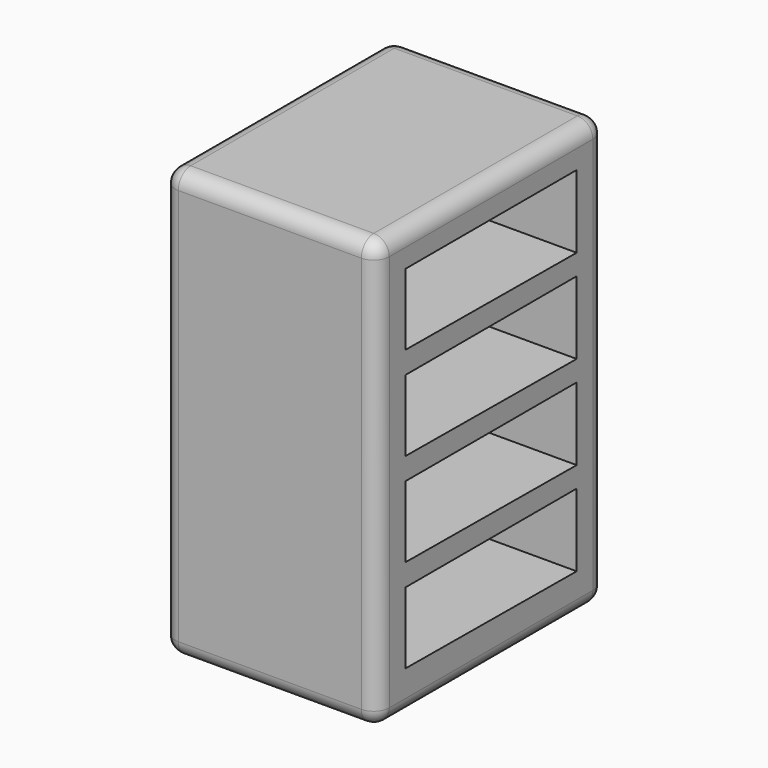
from build123d import *

# Parameters (mm, degrees)
F0_W     = 76.2
F0_H     = 101.6
F1_DEPTH = 152.4
F3_DEPTH = 50.8
F4_R     = 5.5188922036


# Not quite as in the source:
# - a feature names something its author has since deleted; it is built from what else it names


with BuildPart() as f1:
    # F0 (on Top) → F1 (new body)
    with BuildSketch(Plane.XY):
        with Locations((-5.2541131154, 53.4473587833)):
            Rectangle(F0_W, F0_H)
    extrude(amount=-F1_DEPTH)

    # F2 (on face) → F3 (cut)
    with BuildSketch(Plane.YZ.offset(32.8458868846)):
        Polygon((15.3492157235, -137.4566919493), (91.5473587833, -137.988663984), (91.5473587833, -112.0566919493), (15.3492157235, -112.0566919493), align=None)
        Polygon((15.3492157235, -78.7826919493), (15.3492157235, -104.1826919493), (91.5473587833, -104.714663984), (91.5473587833, -78.7826919493), align=None)
        Polygon((15.3492157235, -45.5086919493), (15.3492157235, -70.9086919493), (91.5473587833, -71.440663984), (91.5473587833, -45.5086919493), align=None)
        Polygon((15.3492157235, -12.2346919493), (15.3492157235, -37.6346919493), (91.5473587833, -38.166663984), (91.5473587833, -12.2346919493), align=None)
    extrude(amount=-F3_DEPTH, mode=Mode.SUBTRACT)

    # F4
    f4_edges = [f1.edges().sort_by_distance(p)[0] for p in [
        (-5.254113, 104.247359, 0),
        (-5.254113, 2.647359, 0),
        (-5.254113, 2.647359, -152.4),
        (-5.254113, 104.247359, -152.4),
        (32.845887, 2.647359, -76.2),
        (32.845887, 53.447359, -152.4),
        (32.845887, 104.247359, -76.2),
        (-43.354113, 53.447359, -152.4),
        (-43.354113, 2.647359, -76.2),
        (32.845887, 53.447359, 0),
        (-43.354113, 53.447359, 0),
        (-43.354113, 104.247359, -76.2),
    ]]
    fillet(f4_edges, radius=F4_R)


solid = f1.part
